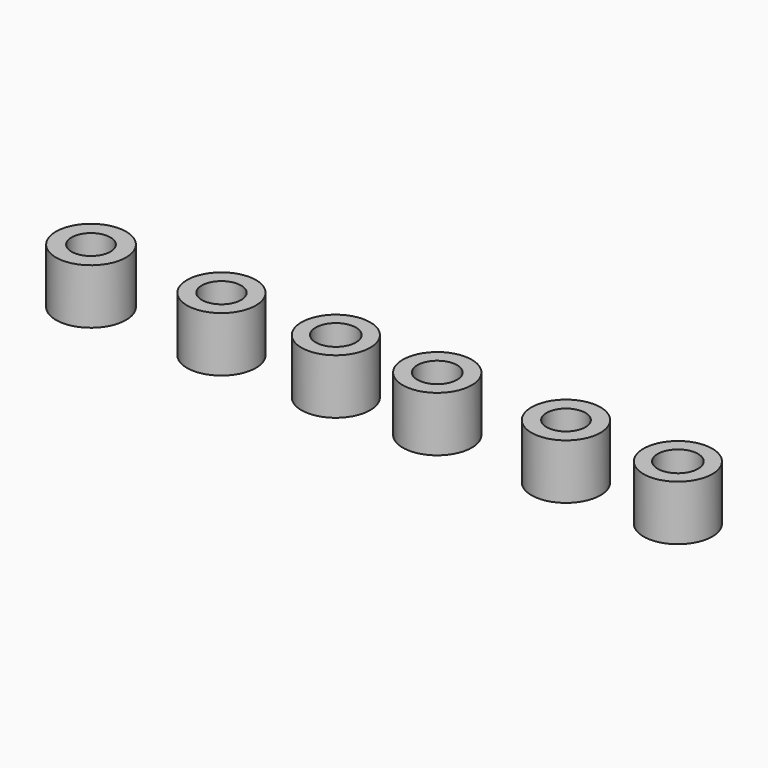
from build123d import *

# Parameters (mm, degrees)
F0_R     = 6.3507220603
F0_R_2   = 3.7192541637
F1_DEPTH = 10.16
F0_R_3   = 6.3619127216
F0_R_4   = 3.6327515113
F0_R_5   = 6.4757284785
F0_R_6   = 3.5860816938
F2_R     = 6.3562234289
F2_R_2   = 3.7276679296
F3_DEPTH = 10.16
F2_R_3   = 6.375345629
F2_R_4   = 3.6654269583
F2_R_5   = 6.3754
F2_R_6   = 3.5851449437


# Not quite as in the source:
# - a feature names something its author has since deleted; it is built from what else it names


with BuildPart() as f1:
    # F0 (on Top) → F1 (new body)
    with BuildSketch(Plane.XY):
        with Locations((-12.6321576536, 0)):
            Circle(F0_R)
        with Locations((-12.6321576536, 0)):
            Circle(F0_R_2, mode=Mode.SUBTRACT)
    extrude(amount=F1_DEPTH)


with BuildPart() as f1b:
    # F0 (on Top) → F1, piece 2 (new body)
    with BuildSketch(Plane.XY):
        with Locations((-33.7451025844, 0)):
            Circle(F0_R_3)
        with Locations((-33.7451025844, 0)):
            Circle(F0_R_4, mode=Mode.SUBTRACT)
    extrude(amount=F1_DEPTH)


with BuildPart() as f1c:
    # F0 (on Top) → F1, piece 3 (new body)
    with BuildSketch(Plane.XY):
        with Locations((-57.8276067972, 0)):
            Circle(F0_R_5)
        with Locations((-57.8276067972, 0)):
            Circle(F0_R_6, mode=Mode.SUBTRACT)
    extrude(amount=F1_DEPTH)


with BuildPart() as f3:
    # F2 (on Top) → F3 (new body)
    with BuildSketch(Plane.XY):
        with Locations((50.5194365978, 0)):
            Circle(F2_R)
        with Locations((50.5194365978, 0)):
            Circle(F2_R_2, mode=Mode.SUBTRACT)
    extrude(amount=F3_DEPTH)


with BuildPart() as f3b:
    # F2 (on Top) → F3, piece 2 (new body)
    with BuildSketch(Plane.XY):
        with Locations((6.093558742, 0)):
            Circle(F2_R_3)
        with Locations((6.093558742, 0)):
            Circle(F2_R_4, mode=Mode.SUBTRACT)
    extrude(amount=F3_DEPTH)


with BuildPart() as f3c:
    # F2 (on Top) → F3, piece 3 (new body)
    with BuildSketch(Plane.XY):
        with Locations((29.8588951446, 0)):
            Circle(F2_R_5)
        with Locations((29.8588951446, 0)):
            Circle(F2_R_6, mode=Mode.SUBTRACT)
    extrude(amount=F3_DEPTH)


solid = Compound([f1.part, f1b.part, f1c.part, f3.part, f3b.part, f3c.part])
